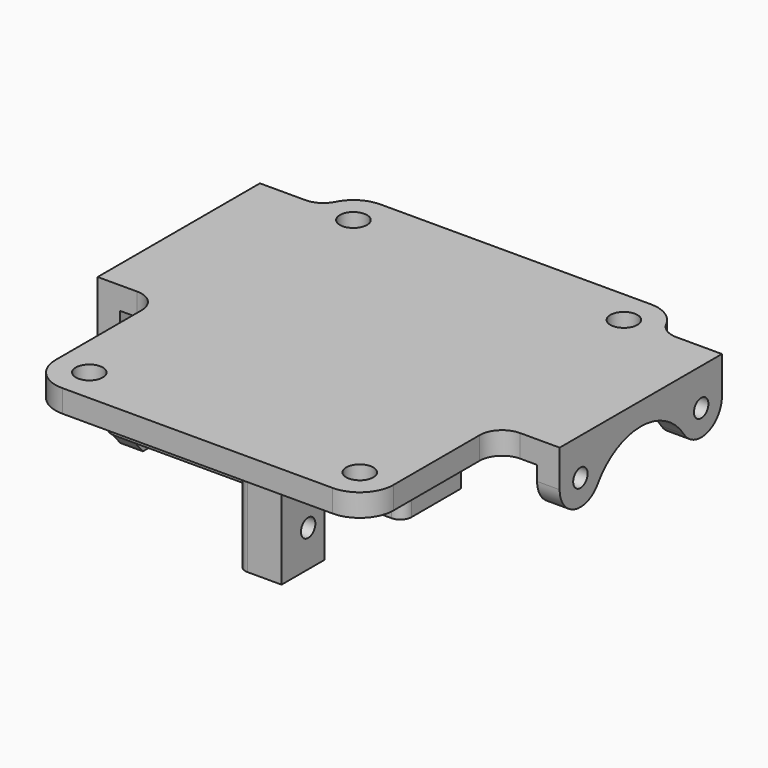
from build123d import *

# Parameters (mm, degrees)
F1_R          = 1.2
F2_DEPTH      = 2
F3_R          = 2
F4_W          = 4
F4_H          = 4.75
F5_DEPTH      = 9
F6_W          = 8.8
F6_H          = 2
F6_W_2        = 2
F6_H_2        = 6.5
F7_DEPTH      = 4
F8_R          = 0.8
F9_DEPTH      = 4
F10_T4_DEPTH  = 2
F10_S5_R      = 0.8
F10_T6_DEPTH  = 3
F10_T10_DEPTH = 6.5
F10_T15_DEPTH = 6.5
F10_T20_DEPTH = 2
F10_S21_R     = 0.8
F10_T22_DEPTH = 3
F10_T27_DEPTH = 6.5
F10_S29_R     = 0.8
F10_T30_DEPTH = 5
F10_T33_DEPTH = 4.5
F10_T40_DEPTH = 4.5
F10_T44_DEPTH = 6.5
F10_S46_R     = 0.8
F10_T47_DEPTH = 5
F10_T49_DEPTH = 6.5
F10_T51_DEPTH = 11.5
F11_W         = 2
F11_H         = 18
F12_DEPTH     = 12
F13_R         = 1.55
F13_R_2       = 0.8
F14_DEPTH     = 2
F15_R         = 0.8
F16_DEPTH     = 2
F18_W         = 20.8
F18_H         = 21.9
F19_DEPTH     = 0.4


# Not quite as in the source:
# - a fillet or chamfer that OpenCascade refuses, or shapes differently, is made with other operations: its cross-section is extruded or revolved along the edge and cut away or added
# - two fillets or chamfers of one size are made in one step


with BuildPart() as f2:
    # F1 (on Top) → F2 (new body)
    with BuildSketch(Plane.XY):
        with BuildLine():
            Line((-4.2895651858, 24.55), (-9.8, 24.55))
            Line((-9.8, 24.55), (-9.8, 6.55))
            Line((-9.8, 6.55), (-4.3, 6.55))
            Line((-4.3, 6.55), (-4.3, -5))
            ThreePointArc((-4.3, -5), (-3.4213203436, -7.1213203436), (-1.3, -8))
            Line((-1.3, -8), (22.7, -8))
            ThreePointArc((22.7, -8), (24.8213203436, -7.1213203436), (25.7, -5))
            Line((25.7, -5), (25.7, 6.55))
            Line((25.7, 6.55), (31.2, 6.55))
            Line((31.2, 6.55), (31.2, 24.55))
            Line((31.2, 24.55), (25.6895651858, 24.55))
            ThreePointArc((25.6895651858, 24.55), (24.7310096012, 26.5079402166), (22.7, 27.3))
            Line((22.7, 27.3), (-1.3, 27.3))
            ThreePointArc((-1.3, 27.3), (-3.3310096012, 26.5079402166), (-4.2895651858, 24.55))
        make_face()
        with Locations((-1.3, -5)):
            Circle(F1_R, mode=Mode.SUBTRACT)
        with Locations((22.7, -5)):
            Circle(F1_R, mode=Mode.SUBTRACT)
        with Locations((-1.3, 24.3)):
            Circle(F1_R, mode=Mode.SUBTRACT)
        with Locations((22.7, 24.3)):
            Circle(F1_R, mode=Mode.SUBTRACT)
    extrude(amount=F2_DEPTH)

    # F3
    f3_edges = [f2.edges().sort_by_distance(p)[0] for p in [
        (-4.289565, 24.55, 1),
        (-4.3, 6.55, 1),
        (25.7, 6.55, 1),
        (25.689565, 24.55, 1),
    ]]
    fillet(f3_edges, radius=F3_R)

    # F4 (on face) → F5 (join)
    with BuildSketch(Plane(origin=(0, 0, 0), x_dir=(1, 0, 0), z_dir=(0, 0, -1))):
        with Locations((13.8, 2.675)):
            Rectangle(F4_W, F4_H)
        with Locations((13.8, -23.975)):
            Rectangle(F4_W, F4_H)
    extrude(amount=F5_DEPTH)

    # F6 (on face) → F7 (join)
    with BuildSketch(Plane(origin=(0, 0, 0), x_dir=(1, 0, 0), z_dir=(0, 0, -1))):
        Polygon((-2.3, -18.3), (-0.3, -18.3), (-0.3, 0.3), (11.8, 0.3), (11.8, 2.3), (-2.3, 2.3), align=None)
        with Locations((7.4, -22.6)):
            Rectangle(F6_W, F6_H)
        with Locations((21.5, -3.25)):
            Rectangle(F6_W_2, F6_H_2)
    extrude(amount=F7_DEPTH)

    # F8 (on face) → F9 (cut, through all)
    with BuildSketch(Plane.YZ.offset(15.8)):
        with Locations((23.4, -5.75)):
            Circle(F8_R)
        with Locations((-2.1, -5.75)):
            Circle(F8_R)
    extrude(amount=-F9_DEPTH, mode=Mode.SUBTRACT)

    # F10: fillet of radius 1 on 10 edges, made by hand


with BuildPart() as f10_tool2:
    # F10_s3 → F10_t4 (new body)
    with BuildSketch(Plane.XZ.offset(0.3)):
        with BuildLine():
            ThreePointArc((11.8, -5), (11.5071067812, -4.2928932188), (10.8, -4))
            Line((10.8, -4), (11.8, -4))
            Line((11.8, -4), (11.8, -5))
        make_face()
    extrude(amount=F10_T4_DEPTH)

    # F10_s5 → F10_t6 (cut, symmetric)
    with BuildSketch(Plane.YZ.offset(11.3)):
        with Locations((-2.1, -5.75)):
            Circle(F10_S5_R)
    extrude(amount=F10_T6_DEPTH, both=True, mode=Mode.SUBTRACT)


with BuildPart() as f2_1:
    add(f2.part)

    # F10_t1: union F10_tool2
    add(f10_tool2.part)


with BuildPart() as f10_tool8:
    # F10_s9 → F10_t10 (new body)
    with BuildSketch(Plane.XY.offset(2.5)):
        with BuildLine():
            ThreePointArc((11.8, -3.3), (11.5071067812, -2.5928932188), (10.8, -2.3))
            Line((10.8, -2.3), (11.8, -2.3))
            Line((11.8, -2.3), (11.8, -3.3))
        make_face()
    extrude(amount=-F10_T10_DEPTH)

    split(bisect_by=Plane.XY.offset(2), keep=Keep.BOTTOM)


with BuildPart() as f2_2:
    add(f2_1.part)

    # F10_t7: union F10_tool8
    add(f10_tool8.part)


with BuildPart() as f10_tool13:
    # F10_s14 → F10_t15 (new body)
    with BuildSketch(Plane.XY.offset(2.5)):
        with BuildLine():
            ThreePointArc((11.8, 24.6), (11.5071067812, 23.8928932188), (10.8, 23.6))
            Line((10.8, 23.6), (11.8, 23.6))
            Line((11.8, 23.6), (11.8, 24.6))
        make_face()
    extrude(amount=-F10_T15_DEPTH)

    split(bisect_by=Plane.XY.offset(2), keep=Keep.BOTTOM)


with BuildPart() as f2_3:
    add(f2_2.part)

    # F10_t12: union F10_tool13
    add(f10_tool13.part)


with BuildPart() as f10_tool18:
    # F10_s19 → F10_t20 (new body)
    with BuildSketch(Plane.XZ.offset(-23.6)):
        with BuildLine():
            ThreePointArc((11.8, -5), (11.5071067812, -4.2928932188), (10.8, -4))
            Line((10.8, -4), (11.8, -4))
            Line((11.8, -4), (11.8, -5))
        make_face()
    extrude(amount=F10_T20_DEPTH)

    # F10_s21 → F10_t22 (cut, symmetric)
    with BuildSketch(Plane.YZ.offset(11.3)):
        with Locations((23.4, -5.75)):
            Circle(F10_S21_R)
    extrude(amount=F10_T22_DEPTH, both=True, mode=Mode.SUBTRACT)


with BuildPart() as f2_4:
    add(f2_3.part)

    # F10_t17: union F10_tool18
    add(f10_tool18.part)


with BuildPart() as f10_tool25:
    # F10_s26 → F10_t27 (new body)
    with BuildSketch(Plane.XY):
        with BuildLine():
            ThreePointArc((11.8, -3.3), (11.5071067812, -2.5928932188), (10.8, -2.3))
            Line((10.8, -2.3), (11.8, -2.3))
            Line((11.8, -2.3), (11.8, -3.3))
        make_face()
    extrude(amount=-F10_T27_DEPTH)

    split(bisect_by=Plane.XY.offset(-4), keep=Keep.BOTTOM)

    # F10_s29 → F10_t30 (cut, symmetric)
    with BuildSketch(Plane.YZ.offset(11.3)):
        with Locations((-2.1, -5.75)):
            Circle(F10_S29_R)
    extrude(amount=F10_T30_DEPTH, both=True, mode=Mode.SUBTRACT)


with BuildPart() as f10_tool31:
    # F10_s32 → F10_t33 (new body)
    with BuildSketch(Plane.XZ.offset(0.3)):
        with BuildLine():
            ThreePointArc((11.8, -5), (11.5071067812, -4.2928932188), (10.8, -4))
            Line((10.8, -4), (11.8, -4))
            Line((11.8, -4), (11.8, -5))
        make_face()
    extrude(amount=F10_T33_DEPTH)

    split(bisect_by=Plane.XZ.offset(2.3), keep=Keep.TOP)


with BuildPart() as f10_tool25_1:
    add(f10_tool25.part)

    # F10_t35: intersect F10_tool31
    add(f10_tool31.part, mode=Mode.INTERSECT)


with BuildPart() as f2_5:
    add(f2_4.part)

    # F10_t23: union F10_tool25
    add(f10_tool25_1.part)


with BuildPart() as f10_tool38:
    # F10_s39 → F10_t40 (new body)
    with BuildSketch(Plane.XZ.offset(-26.1)):
        with BuildLine():
            ThreePointArc((11.8, -5), (11.5071067812, -4.2928932188), (10.8, -4))
            Line((10.8, -4), (11.8, -4))
            Line((11.8, -4), (11.8, -5))
        make_face()
    extrude(amount=F10_T40_DEPTH)

    split(bisect_by=Plane.XZ.offset(-23.6), keep=Keep.BOTTOM)


with BuildPart() as f10_tool42:
    # F10_s43 → F10_t44 (new body)
    with BuildSketch(Plane.XY):
        with BuildLine():
            ThreePointArc((11.8, 24.6), (11.5071067812, 23.8928932188), (10.8, 23.6))
            Line((10.8, 23.6), (11.8, 23.6))
            Line((11.8, 23.6), (11.8, 24.6))
        make_face()
    extrude(amount=-F10_T44_DEPTH)

    split(bisect_by=Plane.XY.offset(-4), keep=Keep.BOTTOM)

    # F10_s46 → F10_t47 (cut, symmetric)
    with BuildSketch(Plane.YZ.offset(11.3)):
        with Locations((23.4, -5.75)):
            Circle(F10_S46_R)
    extrude(amount=F10_T47_DEPTH, both=True, mode=Mode.SUBTRACT)


with BuildPart() as f10_tool38_1:
    add(f10_tool38.part)

    # F10_t48: intersect F10_tool42
    add(f10_tool42.part, mode=Mode.INTERSECT)


with BuildPart() as f2_6:
    add(f2_5.part)

    # F10_t36: union F10_tool38
    add(f10_tool38_1.part)

    # F10_s50 → F10_t49 (cut)
    with BuildSketch(Plane.XY.offset(-6.5)):
        with BuildLine():
            ThreePointArc((-1.3, -2.3), (-2.0071067812, -2.0071067812), (-2.3, -1.3))
            Line((-2.3, -1.3), (-2.3, -2.3))
            Line((-2.3, -2.3), (-1.3, -2.3))
        make_face()
        with BuildLine():
            ThreePointArc((-2.3, 17.3), (-2.0071067812, 18.0071067812), (-1.3, 18.3))
            Line((-1.3, 18.3), (-2.3, 18.3))
            Line((-2.3, 18.3), (-2.3, 17.3))
        make_face()
        with BuildLine():
            ThreePointArc((3, 22.6), (3.2928932188, 23.3071067812), (4, 23.6))
            Line((4, 23.6), (3, 23.6))
            Line((3, 23.6), (3, 22.6))
        make_face()
        with BuildLine():
            ThreePointArc((21.5, 0), (22.2071067812, 0.2928932188), (22.5, 1))
            Line((22.5, 1), (22.5, 0))
            Line((22.5, 0), (21.5, 0))
        make_face()
    extrude(amount=F10_T49_DEPTH, mode=Mode.SUBTRACT)

    # F10_s52 → F10_t51 (cut)
    with BuildSketch(Plane.XY.offset(-11.5)):
        with BuildLine():
            ThreePointArc((11.8, 25.35), (12.0928932188, 26.0571067812), (12.8, 26.35))
            Line((12.8, 26.35), (11.8, 26.35))
            Line((11.8, 26.35), (11.8, 25.35))
        make_face()
        with BuildLine():
            ThreePointArc((12.8, -5.05), (12.0928932188, -4.7571067812), (11.8, -4.05))
            Line((11.8, -4.05), (11.8, -5.05))
            Line((11.8, -5.05), (12.8, -5.05))
        make_face()
    extrude(amount=F10_T51_DEPTH, mode=Mode.SUBTRACT)

    # F11 (on face) → F12 (join)
    with BuildSketch(Plane(origin=(0, 0, 0), x_dir=(1, 0, 0), z_dir=(0, 0, -1))):
        with Locations((-8.8, -15.55)):
            Rectangle(F11_W, F11_H)
        with Locations((30.2, -15.55)):
            Rectangle(F11_W, F11_H)
    extrude(amount=F12_DEPTH)

    # F13 (on face) → F14 (cut, through all)
    with BuildSketch(Plane(origin=(-9.8, 0, 0), x_dir=(0, -1, 0), z_dir=(-1, 0, 0))):
        with Locations((-15.55, -5.75)):
            Circle(F13_R)
        with Locations((-21.55, -5.75)):
            Circle(F13_R_2)
        with Locations((-9.55, -5.75)):
            Circle(F13_R_2)
        with BuildLine():
            ThreePointArc((-22.0259169235, -12), (-23.8951558497, -9.1202186642), (-24.55, -5.75))
            Line((-24.55, -5.75), (-24.55, -12))
            Line((-24.55, -12), (-22.0259169235, -12))
        make_face()
        with BuildLine():
            ThreePointArc((-6.55, -5.75), (-7.2048441503, -9.1202186642), (-9.0740830765, -12))
            Line((-9.0740830765, -12), (-6.55, -12))
            Line((-6.55, -12), (-6.55, -5.75))
        make_face()
    extrude(amount=-F14_DEPTH, mode=Mode.SUBTRACT)

    # F15 (on face) → F16 (cut, through all)
    with BuildSketch(Plane.YZ.offset(31.2)):
        with BuildLine():
            ThreePointArc((24.55, -1.2876575658), (22.9160115829, -3.4891181199), (20.3357142857, -2.562612547))
            ThreePointArc((20.3357142857, -2.562612547), (15.55, 0), (10.7642857143, -2.562612547))
            ThreePointArc((10.7642857143, -2.562612547), (8.1839884171, -3.4891181199), (6.55, -1.2876575658))
            Line((6.55, -1.2876575658), (6.55, -12))
            Line((6.55, -12), (24.55, -12))
            Line((24.55, -12), (24.55, -1.2876575658))
        make_face()
        with Locations((8.85, -1.2876575658)):
            Circle(F15_R)
        with Locations((22.25, -1.2876575658)):
            Circle(F15_R)
    extrude(amount=-F16_DEPTH, mode=Mode.SUBTRACT)

    # F18 (on face) → F19 (cut)
    with BuildSketch(Plane(origin=(0, 0, 0), x_dir=(1, 0, 0), z_dir=(0, 0, -1))):
        with Locations((10.1, -10.65)):
            Rectangle(F18_W, F18_H)
    extrude(amount=-F19_DEPTH, mode=Mode.SUBTRACT)


solid = f2_6.part
